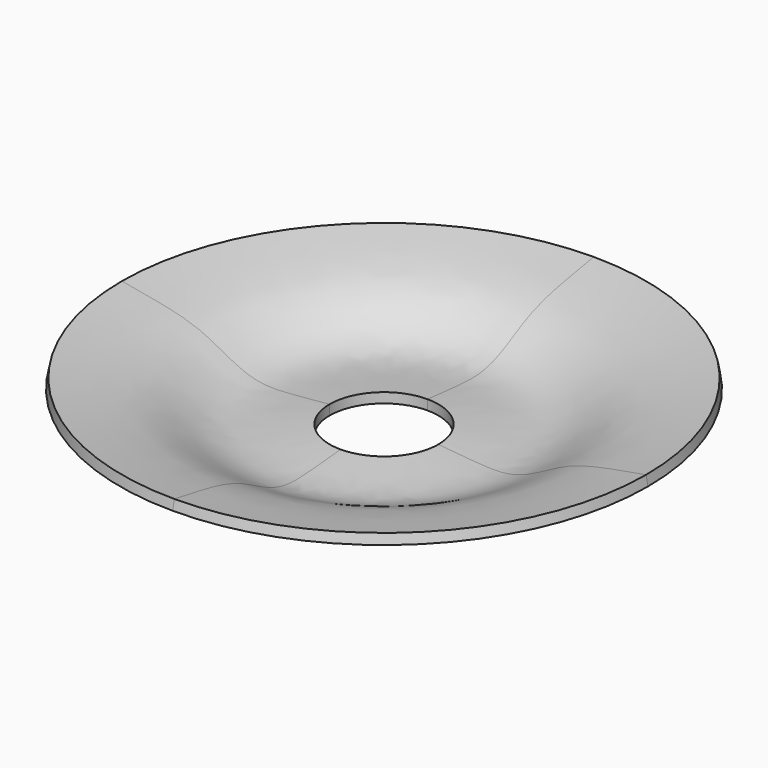
from build123d import *

# Parameters (mm, degrees)
F1_ANGLE        = 90
F1_COPIES_COUNT = 4
F2_R            = 19.3178847041
F3_DEPTH        = 12.5


# Not quite as in the source:
# - a feature of the source that left no trace in its solid (it failed there, or was rolled back) is left out
# - the dataset's text gives a spline's control points without its knots; the knots are read off the source's solid
# - a pattern or mirror of a feature is missing from the dataset's text; its kind, count and spacing are read off the source's solid


with BuildPart() as f1:
    # F0 (on Front) → F1 (revolve)
    with BuildSketch(Plane.XZ):
        with BuildLine():
            add(Edge.make_bspline(
                [(0.535384993, 0.1223555221), (17.2094367636, 3.8394536298), (43.2929624479, -5.465311782), (64.2545376437, 11.4596925852), (81.7273993655, 13.6582770662), (93.1396260858, 15.7730262727)],
                knots=[0.004141275, 0.004141275, 0.004141275, 0.004141275, 0.3914803814, 0.6772663946, 1, 1, 1, 1], degree=3))
            Line((0.535384993, 0.1223555221), (0.474259215, -3.4347528534))
            Line((0.474259215, -3.4347528534), (0.8043280011, -3.4347528534))
            add(Edge.make_bspline(
                [(0.8043280011, -3.4347528534), (3.3148291149, -2.8468600912), (8.2742920499, -2.1143351467), (15.5332184992, -1.9868717443), (22.5825008916, -2.4781703416), (28.248732939, -3.0969025959), (32.6463450247, -3.5216344609), (35.8777622406, -3.7523528033), (39.0462368261, -3.838931027), (41.6353513211, -3.7390833353), (43.6825461889, -3.5194285423), (45.6918972373, -3.1953102754), (48.0788038091, -2.6179690834), (50.7700150604, -1.7083774784), (53.3020669479, -0.643306801), (55.7005846476, 0.5201483357), (57.9922146811, 1.7293684368), (60.2039145986, 2.9362082665), (62.3608906754, 4.0964681393), (64.1325757078, 4.9908391226), (65.5452849821, 5.6448511365), (66.9605812541, 6.2523714935), (68.7937846142, 6.9489329742), (71.0931629092, 7.695431129), (73.5021272144, 8.3680692714), (76.8661994201, 9.1856648058), (81.3678679034, 10.0966139075), (87.2697497294, 11.1392380289), (91.5514001783, 11.890991348), (93.7823810236, 12.3044045309)],
                knots=[0, 0, 0, 0, 0.0625, 0.125, 0.1875, 0.25, 0.28125, 0.3125, 0.34375, 0.375, 0.390625, 0.40625, 0.4375, 0.46875, 0.5, 0.53125, 0.5625, 0.59375, 0.625, 0.65625, 0.671875, 0.6875, 0.71875, 0.75, 0.78125, 0.8125, 0.875, 0.9375, 1, 1, 1, 1], degree=3))
            Line((93.7823810236, 12.3044045309), (93.1396260858, 15.7730262727))
        make_face()
    revolve(axis=Axis((0, 0, -1.7173764267), (0, 0, -1)), revolution_arc=F1_ANGLE)


with BuildPart() as f1_copies_1:
    # F1_copies: instance of F1
    add(f1.part.rotate(Axis((0, 0, 0), (0, 0, 1)), 1 * 360 / F1_COPIES_COUNT))


with BuildPart() as f1_copies_2:
    # F1_copies: instance of F1
    add(f1.part.rotate(Axis((0, 0, 0), (0, 0, 1)), 2 * 360 / F1_COPIES_COUNT))


with BuildPart() as f1_copies_3:
    # F1_copies: instance of F1
    add(f1.part.rotate(Axis((0, 0, 0), (0, 0, 1)), 3 * 360 / F1_COPIES_COUNT))


with BuildPart() as f3_tool:
    # F2 (on Top) → F3 (new body, symmetric)
    with BuildSketch(Plane.XY):
        Circle(F2_R)
    extrude(amount=F3_DEPTH, both=True)


with BuildPart() as f1_1:
    add(f1.part)

    # F3: cut by f3_tool
    add(f3_tool.part, mode=Mode.SUBTRACT)


with BuildPart() as f1_copies_1_1:
    add(f1_copies_1.part)

    # F3: cut by f3_tool
    add(f3_tool.part, mode=Mode.SUBTRACT)


with BuildPart() as f1_copies_2_1:
    add(f1_copies_2.part)

    # F3: cut by f3_tool
    add(f3_tool.part, mode=Mode.SUBTRACT)


with BuildPart() as f1_copies_3_1:
    add(f1_copies_3.part)

    # F3: cut by f3_tool
    add(f3_tool.part, mode=Mode.SUBTRACT)


solid = Compound([f1_1.part, f1_copies_1_1.part, f1_copies_2_1.part, f1_copies_3_1.part])
